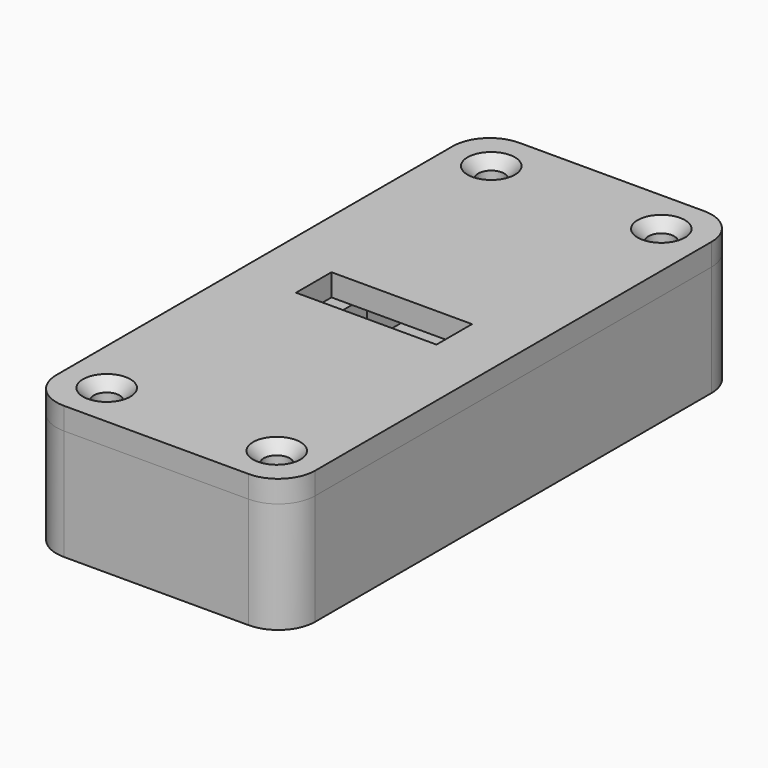
from build123d import *

# Parameters (mm, degrees)
F0_W            = 35
F0_H            = 77
F1_DEPTH        = 15
F2_W            = 31.4
F2_H            = 53
F3_DEPTH        = 13
F4_W            = 12
F4_H            = 3
F5_DEPTH        = 25
F7_W            = 35
F7_H            = 77
F8_DEPTH        = 3
F11_D           = 3.5
F11_CSINK_D     = 6.4
F11_CSINK_ANGLE = 90
F12_R           = 5
F12_2_R         = 5
F13_W           = 31
F13_H           = 18
F14_DEPTH       = 12.7
F16_DEPTH       = 18
F9_W            = 19
F9_H            = 6
F17_DEPTH       = 3


# Not quite as in the source:
# - a feature names something its author has since deleted; it is built from what else it names


with BuildPart() as f1:
    # F0 (on Top) → F1 (new body)
    with BuildSketch(Plane.XY):
        with Locations((17.5, 38.5)):
            Rectangle(F0_W, F0_H)
    extrude(amount=F1_DEPTH)

    # F2 (on face) → F3 (cut)
    with BuildSketch(Plane.XY.offset(15)):
        with Locations((17.5, 38.5)):
            Rectangle(F2_W, F2_H)
    extrude(amount=-F3_DEPTH, mode=Mode.SUBTRACT)

    # F4 (on face) → F5 (cut)
    with BuildSketch(Plane.XZ.offset(-65)):
        with Locations((17.7, 13.5)):
            Rectangle(F4_W, F4_H)
    extrude(amount=-F5_DEPTH, mode=Mode.SUBTRACT)

    # F12
    f12_edges = [f1.edges().sort_by_distance(p)[0] for p in [
        (35, 77, 7.5),
        (0, 77, 7.5),
        (35, 0, 7.5),
        (0, 0, 7.5),
    ]]
    fillet(f12_edges, radius=F12_R)


with BuildPart() as f8:
    # F7 (on face) → F8 (new body)
    with BuildSketch(Plane.XY.offset(15)):
        with Locations((17.5, 38.5)):
            Rectangle(F7_W, F7_H)
    extrude(amount=F8_DEPTH)

    # F11 (through all)
    with Locations(Plane.XY.offset(18)):
        with Locations((6, 71), (29, 71), (29, 6), (6, 6)):
            CounterSinkHole(F11_D / 2, F11_CSINK_D / 2, counter_sink_angle=F11_CSINK_ANGLE)

    # F12#2
    f12_2_edges = [f8.edges().sort_by_distance(p)[0] for p in [
        (35, 77, 16.5),
        (0, 77, 16.5),
        (35, 0, 16.5),
        (0, 0, 16.5),
    ]]
    fillet(f12_2_edges, radius=F12_2_R)

    # F9 (on face) → F17 (cut, through all)
    with BuildSketch(Plane(origin=(0, 0, 15), x_dir=(1, 0, 0), z_dir=(0, 0, -1))):
        with Locations((17.5, -38.5)):
            Rectangle(F9_W, F9_H)
    extrude(amount=-F17_DEPTH, mode=Mode.SUBTRACT)


with BuildPart() as f14:
    # F13 (on face) → F14 (new body, through all)
    with BuildSketch(Plane.XY.offset(2)):
        with Locations((17.5, 35.4918729663)):
            Rectangle(F13_W, F13_H)
    extrude(amount=F14_DEPTH)

    # F15 (on face) → F16 (cut, through all)
    with BuildSketch(Plane(origin=(0, 44.4918729663, 0), x_dir=(-1, 0, 0), z_dir=(0, 1, 0))):
        Polygon((-24.6, 14.7), (-24.6, 10), (-24.6, 6.55), (-25.35, 6.55), (-25.35, 4.7), (-24.6, 4.7), (-24.6, 3.5), (-10.4, 3.5), (-10.4, 5), (-9.65, 5), (-9.65, 6.85), (-10.4, 6.85), (-10.4, 10), (-10.4, 14.7), align=None)
    extrude(amount=-F16_DEPTH, mode=Mode.SUBTRACT)


solid = Compound([f1.part, f8.part, f14.part])
